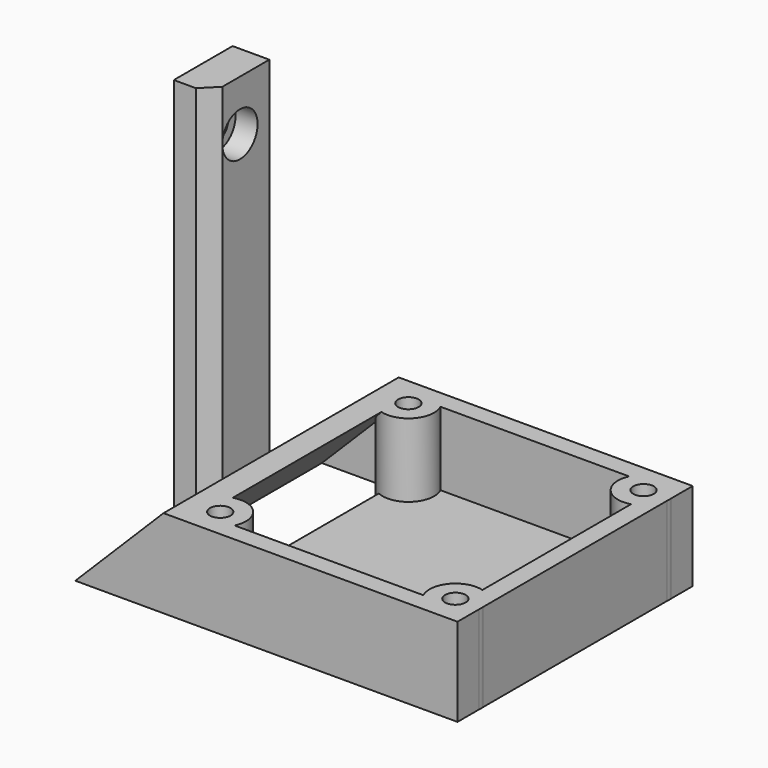
from build123d import *

# Parameters (mm, degrees)
F1_DEPTH  = 40
F2_T      = -2.5
F3_R      = 3.5
F4_DEPTH  = 12
F5_R      = 1.4
F6_DEPTH  = 12.001
F7_W      = 38.9644660941
F7_H      = 40
F8_DEPTH  = 2
F9_SIZE   = 1.99999
F12_DEPTH = 5
F13_R     = 1.75
F14_DEPTH = 12.001
F15_R     = 3
F16_DEPTH = 3
F17_SIZE  = 1.99999


# Not quite as in the source:
# - a fillet or chamfer is up to 0.001 mm smaller than in the source, because OpenCascade refuses the exact size


with BuildPart() as f1:
    # F0 (on Front) → F1 (new body)
    with BuildSketch(Plane.XZ):
        Polygon((12, 12), (0, 0), (52, 0), (52, 12), align=None)
    extrude(amount=F1_DEPTH)

    # F2
    f2_openings = [f1.faces().sort_by_distance(p)[0] for p in [
        (32, -20, 12),
        (26, -20, 0),
    ]]
    offset(amount=F2_T, openings=f2_openings, kind=Kind.INTERSECTION)

    # F3 (on face) → F4 (join, through all)
    with BuildSketch(Plane.XY.offset(12)):
        with Locations((16.517766953, -36)):
            Circle(F3_R)
        with Locations((48.517766953, -36)):
            Circle(F3_R)
        with Locations((48.517766953, -4)):
            Circle(F3_R)
        with Locations((16.517766953, -4)):
            Circle(F3_R)
    extrude(amount=-F4_DEPTH)

    # F5 (on face) → F6 (cut, through all)
    with BuildSketch(Plane.XY.offset(12)):
        with Locations((16.517766953, -4)):
            Circle(F5_R)
        with Locations((48.517766953, -4)):
            Circle(F5_R)
        with Locations((48.517766953, -36)):
            Circle(F5_R)
        with Locations((16.517766953, -36)):
            Circle(F5_R)
    extrude(amount=-F6_DEPTH, mode=Mode.SUBTRACT)

    # F7 (on face) → F8 (join)
    with BuildSketch(Plane(origin=(0, 0, 0), x_dir=(1, 0, 0), z_dir=(0, 0, -1))):
        with Locations((32.517766953, 20)):
            Rectangle(F7_W, F7_H)
    extrude(amount=-F8_DEPTH)

    # F9 (size 2 in the source; OpenCascade refuses exactly that, so slightly less here)
    f9_edges = [f1.edges().sort_by_distance(p)[0] for p in [
        (13.035534, -20, 2),
    ]]
    chamfer(f9_edges, length=F9_SIZE)

    # F11 (on offset) → F12 (join, symmetric)
    with BuildSketch(Plane.XZ.offset(27)):
        Polygon((7, 59), (7, 7), (12, 12), (12, 59), align=None)
    extrude(amount=F12_DEPTH, both=True)

    # F13 (on face) → F14 (cut, through all)
    with BuildSketch(Plane.YZ.offset(12)):
        with Locations((-27, 52.1)):
            Circle(F13_R)
    extrude(amount=-F14_DEPTH, mode=Mode.SUBTRACT)

    # F15 (on face) → F16 (cut)
    with BuildSketch(Plane.YZ.offset(12)):
        with Locations((-27, 52.1)):
            Circle(F15_R)
    extrude(amount=-F16_DEPTH, mode=Mode.SUBTRACT)

    # F17 (size 2 in the source; OpenCascade refuses exactly that, so slightly less here)
    f17_edges = [f1.edges().sort_by_distance(p)[0] for p in [
        (12, -32, 35.5),
    ]]
    chamfer(f17_edges, length=F17_SIZE)


solid = f1.part
